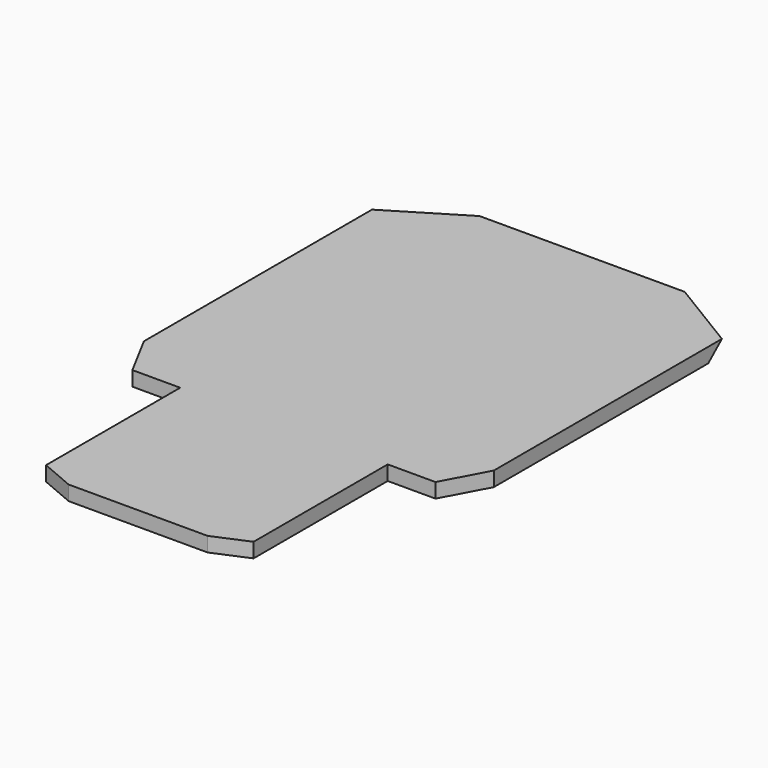
from build123d import *

# Parameters (mm, degrees)
F1_DEPTH    = 3
F2_T1_DEPTH = 42.4243909264
F2_T3_DEPTH = 68.8811967359
F2_T5_DEPTH = 42.4243909264


# Not quite as in the source:
# - a fillet or chamfer that OpenCascade refuses, or shapes differently, is made with other operations: its cross-section is extruded or revolved along the edge and cut away or added


with BuildPart() as f1:
    # F0 (on Top) → F1 (new body)
    with BuildSketch(Plane.XY):
        Polygon((50.666670315, 47.8041956116), (7.5023034588, 47.8041956116), (-6.7788518712, 39.1329097454), (-6.7788518712, -21.6580425002), (-1.982757669, -30.5968765852), (7.8172552019, -30.5968765852), (7.8172552019, -64.9542560763), (14.8365469649, -67.9511922197), (43.3324268088, -67.9511922197), (50.3517185719, -64.9542560763), (50.3517185719, -30.5968765852), (60.1517314427, -30.5968765852), (64.9478256449, -21.6580425002), (64.9478256449, 39.1329097454), align=None)
    extrude(amount=F1_DEPTH)

    # F2: chamfer of 5 on 3 edges, made by hand

    # F2_s2 → F2_t1 (cut)
    with BuildSketch(Plane(origin=(41.0836527068, -24.9453275187, 0), x_dir=(0, 0, 1), z_dir=(-0.8547719975, 0.5190036919, 0))):
        Polygon((5, 67.1578767244), (0, 62.1578767244), (0, 67.1578767244), align=None)
    extrude(amount=F2_T1_DEPTH, mode=Mode.SUBTRACT)

    # F2_s4 → F2_t3 (cut)
    with BuildSketch(Plane.YZ.offset(-5.3561114811)):
        Polygon((47.8041956116, 5), (42.8041956116, 0), (47.8041956116, 0), align=None)
    extrude(amount=F2_T3_DEPTH, mode=Mode.SUBTRACT)

    # F2_s6 → F2_t5 (cut)
    with BuildSketch(Plane(origin=(37.6798265821, 22.8785795082, 0), x_dir=(0, 0, 1), z_dir=(-0.8547719975, -0.5190036919, 0))):
        Polygon((5, 36.9679645806), (0, 31.9679645806), (0, 36.9679645806), align=None)
    extrude(amount=F2_T5_DEPTH, mode=Mode.SUBTRACT)


solid = f1.part
